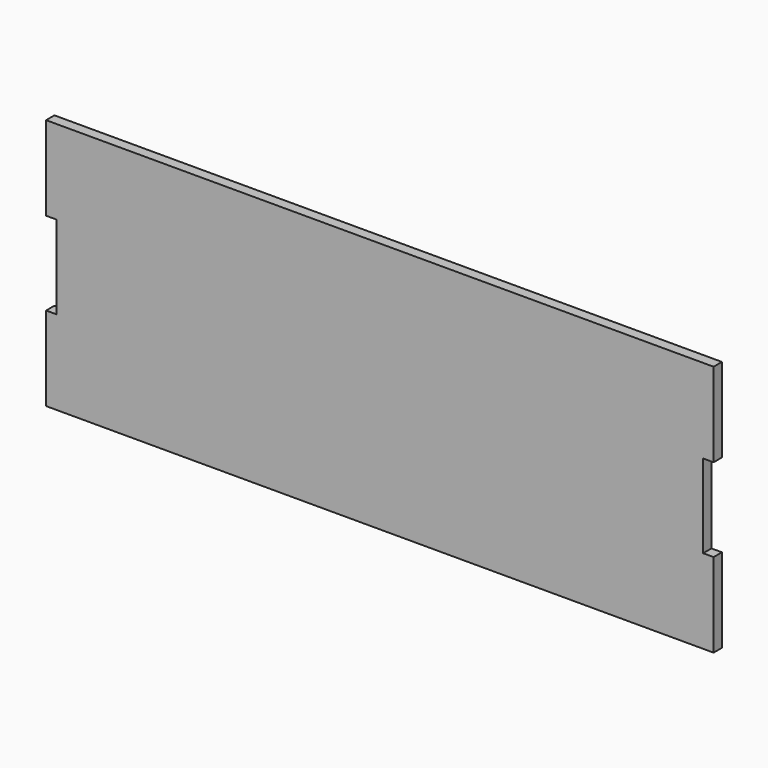
from build123d import *

# Parameters (mm, degrees)
F1_DEPTH = 3.175


# Not quite as in the source:
# - a length typed as a fraction of an inch, garbled in the dataset ("3 / 203.2 mm" for 3/8 in), is restored


with BuildPart() as f1:
    # F0 (on Front) → F1 (new body)
    with BuildSketch(Plane.XZ):
        Polygon((-101.6, 39.6875), (-101.6, 14.2875), (-101.6, 14.1605), (-101.6, 14.0716), (-98.425, 14.0716), (-98.425, 1.3716), (-98.425, -11.3284), (-101.6, -11.3284), (-101.6, -14.1605), (-101.6, -14.2875), (-101.6, -36.9443), (0, -36.9443), (101.6, -36.9443), (101.6, -14.2875), (101.6, -14.1605), (101.6, -11.3284), (98.425, -11.3284), (98.425, 1.3716), (98.425, 14.0716), (101.6, 14.0716), (101.6, 14.1605), (101.6, 14.2875), (101.6, 39.6875), (0, 39.6875), align=None)
    extrude(amount=F1_DEPTH)


solid = f1.part
